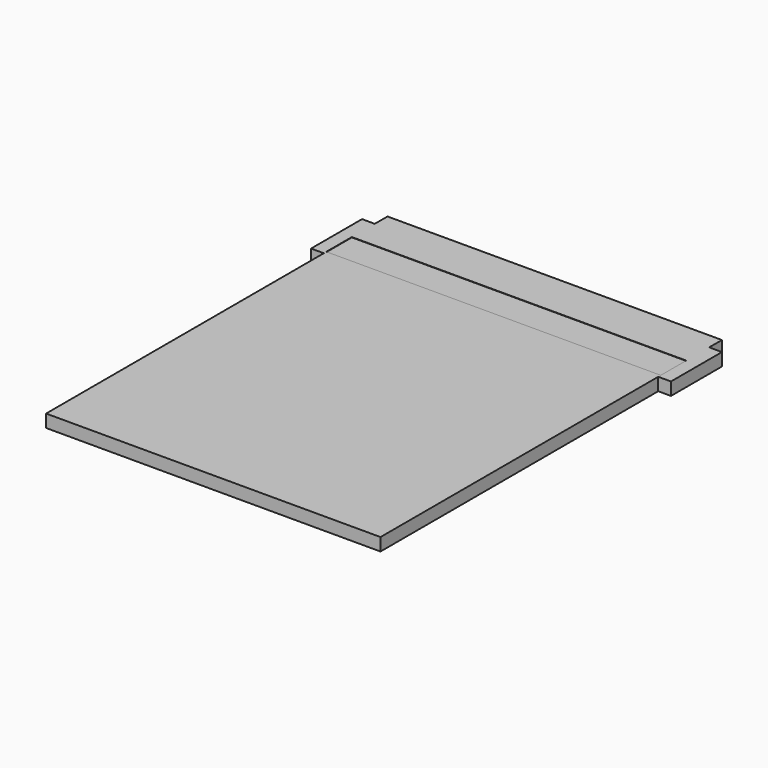
from build123d import *

# Parameters (mm, degrees)
F1_DEPTH = 4
F2_W     = 105
F2_H     = 10
F3_DEPTH = 0.1


# Not quite as in the source:
# - a feature names something its author has since deleted; it is built from what else it names


with BuildPart() as f1:
    # F0 (on Top) → F1 (new body)
    with BuildSketch(Plane.XY):
        Polygon((-52.5, -64.5), (52.5, -64.5), (52.5, 44.5), (56.5, 44.5), (56.5, 64.5), (52.5, 64.5), (52.5, 69.5), (-52.5, 69.5), (-52.5, 64.5), (-56.5, 64.5), (-56.5, 44.5), (-52.5, 44.5), align=None)
    extrude(amount=F1_DEPTH)

    # F2 (on face) → F3 (cut)
    with BuildSketch(Plane.XY.offset(4)):
        with Locations((0, 50.5)):
            Rectangle(F2_W, F2_H)
    extrude(amount=-F3_DEPTH, mode=Mode.SUBTRACT)


solid = f1.part
